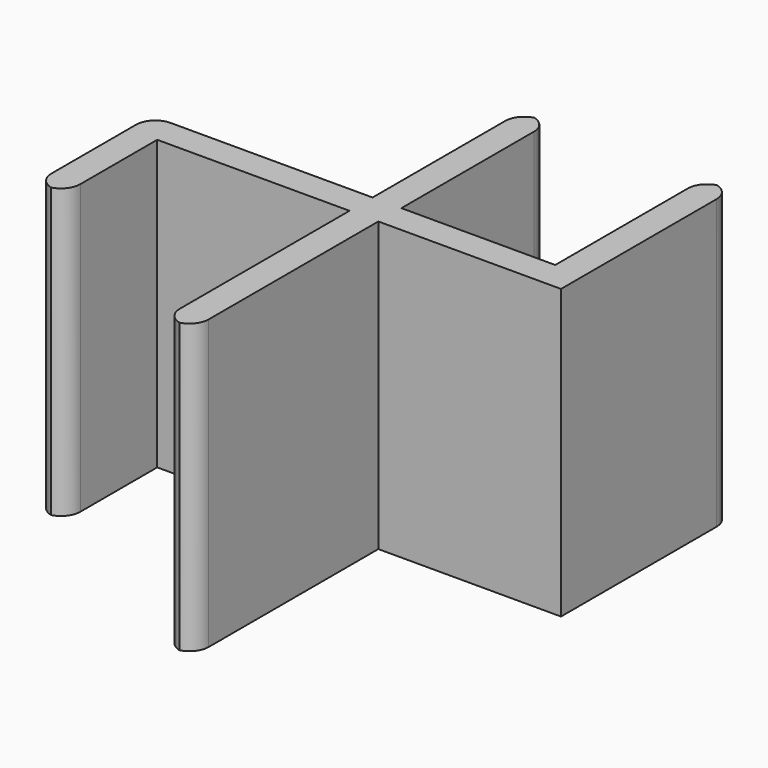
from build123d import *

# Parameters (mm, degrees)
F1_DEPTH    = 30
F2_T1_DEPTH = 40
F3_T1_DEPTH = 40
F4_T1_DEPTH = 40


# Not quite as in the source:
# - a fillet or chamfer that OpenCascade refuses, or shapes differently, is made with other operations: its cross-section is extruded or revolved along the edge and cut away or added


with BuildPart() as f1:
    # F0 (on Top) → F1 (new body)
    with BuildSketch(Plane.XY):
        Polygon((-20, 3), (-23, 3), (-23, -12), (-20, -12), (-20, 0), (0, 0), (0, -12), (0, -24.0508113056), (3, -24.0508113056), (3, -12), (3, 0), (19, 0), (22, 0), (22, 22.2248057965), (19, 22.2248057965), (19, 3), (3, 3), (3, 22.2248057965), (0, 22.2248057965), (0, 3), align=None)
    extrude(amount=F1_DEPTH)

    # F2: fillet of radius 2 on 2 edges, made by hand

    # F2_s2 → F2_t1 (cut)
    with BuildSketch(Plane.XY.offset(-5)):
        with BuildLine():
            ThreePointArc((2, -24.0508113056), (0.5857864376, -23.465024868), (0, -22.0508113056))
            Line((0, -22.0508113056), (0, -24.0508113056))
            Line((0, -24.0508113056), (2, -24.0508113056))
        make_face()
        with BuildLine():
            ThreePointArc((3, -22.0508113056), (2.4142135624, -23.465024868), (1, -24.0508113056))
            Line((1, -24.0508113056), (3, -24.0508113056))
            Line((3, -24.0508113056), (3, -22.0508113056))
        make_face()
    extrude(amount=F2_T1_DEPTH, mode=Mode.SUBTRACT)

    # F3: fillet of radius 2 on 2 edges, made by hand

    # F3_s2 → F3_t1 (cut)
    with BuildSketch(Plane.XY.offset(-5)):
        with BuildLine():
            ThreePointArc((-23, -10), (-22.4142135624, -11.4142135624), (-21, -12))
            Line((-21, -12), (-23, -12))
            Line((-23, -12), (-23, -10))
        make_face()
        with BuildLine():
            ThreePointArc((-22, -12), (-20.5857864376, -11.4142135624), (-20, -10))
            Line((-20, -10), (-20, -12))
            Line((-20, -12), (-22, -12))
        make_face()
    extrude(amount=F3_T1_DEPTH, mode=Mode.SUBTRACT)

    # F4: fillet of radius 2 on 5 edges, made by hand

    # F4_s2 → F4_t1 (cut)
    with BuildSketch(Plane.XY.offset(-5)):
        with BuildLine():
            ThreePointArc((-21, 3), (-22.4142135624, 2.4142135624), (-23, 1))
            Line((-23, 1), (-23, 3))
            Line((-23, 3), (-21, 3))
        make_face()
        with BuildLine():
            ThreePointArc((0, 20.2248057965), (0.5857864376, 21.6390193588), (2, 22.2248057965))
            Line((2, 22.2248057965), (0, 22.2248057965))
            Line((0, 22.2248057965), (0, 20.2248057965))
        make_face()
        with BuildLine():
            ThreePointArc((19, 20.2248057965), (19.5857864376, 21.6390193588), (21, 22.2248057965))
            Line((21, 22.2248057965), (19, 22.2248057965))
            Line((19, 22.2248057965), (19, 20.2248057965))
        make_face()
        with BuildLine():
            ThreePointArc((1, 22.2248057965), (2.4142135624, 21.6390193588), (3, 20.2248057965))
            Line((3, 20.2248057965), (3, 22.2248057965))
            Line((3, 22.2248057965), (1, 22.2248057965))
        make_face()
        with BuildLine():
            ThreePointArc((20, 22.2248057965), (21.4142135624, 21.6390193588), (22, 20.2248057965))
            Line((22, 20.2248057965), (22, 22.2248057965))
            Line((22, 22.2248057965), (20, 22.2248057965))
        make_face()
    extrude(amount=F4_T1_DEPTH, mode=Mode.SUBTRACT)


solid = f1.part
